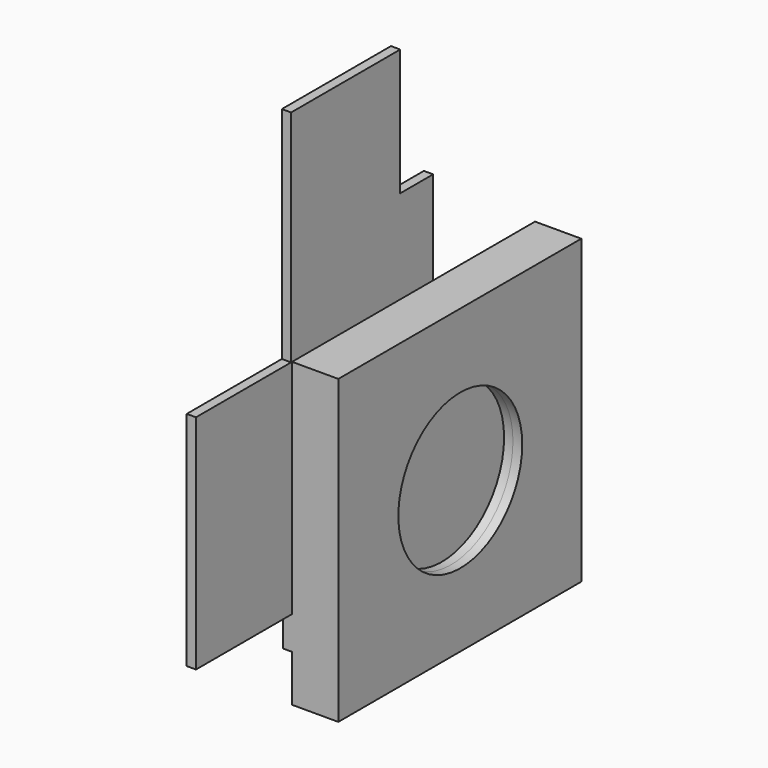
from build123d import *

# Parameters (mm, degrees)
F0_W      = 227.177798748
F0_H      = 67.4825310707
F0_W_2    = 7.6686143875
F0_W_3    = 40.7849550247
F0_H_2    = 19.1998630762
F1_DEPTH  = 25.4
F2_W      = 713.7889862061
F2_H      = 722.4479019642
F3_DEPTH  = 10751.3055801392
F5_W      = 833.6800336838
F5_H      = 828.9024829865
F6_DEPTH  = 25.4
F7_W      = 833.6800336838
F7_H      = 828.9024829865
F7_R      = 213.8106585198
F8_DEPTH  = 25.4
F9_W      = 805.6761920452
F9_H      = 828.9024829865
F9_R      = 212.5191058953
F9_W_2    = 28.0038416386
F10_DEPTH = 25.4
F11_W     = 833.6800336838
F11_H     = 828.9024829865
F11_R     = 151.5456161356
F12_DEPTH = 25.4
F13_W     = 680.4287135601
F13_H     = 667.77536273
F13_R     = 210.9258695705
F14_DEPTH = 25.4
F15_W     = 153.2513201237
F15_H     = 667.77536273
F16_DEPTH = 25.4
F17_W     = 371.1061030626
F17_H     = 256.3967704773
F17_W_2   = 32.0261418819
F17_H_2   = 25.0417590141
F17_W_3   = 119.3500384688
F17_H_3   = 111.177533865
F18_DEPTH = 25.4


with BuildPart() as f1:
    # F0 (on Right) → F1 (new body)
    with BuildSketch(Plane.YZ):
        Polygon((-598.1872081757, 183.7075799704), (-598.1872081757, 196.1238980293), (-605.8558225632, 196.1238980293), (-605.8558225632, 145.6781327724), (-598.1872081757, 145.6781327724), align=None)
        Polygon((-605.8558225632, 196.1238980293), (-598.1872081757, 196.1238980293), (-598.1872081757, 401.8925428391), (-605.8558225632, 401.8925428391), (-605.8558225632, 215.3237611055), align=None)
        Polygon((-1197.3617076874, 196.1238980293), (-605.8558225632, 196.1238980293), (-605.8558225632, 215.3237611055), (-1548.1258630753, 215.3237611055), (-1548.1258630753, 196.1238980293), align=None)
        Polygon((698.481798172, 183.7075799704), (-598.1872081757, 183.7075799704), (-598.1872081757, 145.6781327724), (-598.1872081757, 78.1956017017), (-598.1872081757, 8.7382793427), (698.481798172, 8.7382793427), align=None)
        Polygon((-1197.3617076874, 145.6781327724), (-1197.3617076874, 196.1238980293), (-1548.1258630753, 196.1238980293), (-1548.1258630753, 78.1956017017), (-833.0336213112, 78.1956017017), (-833.0336213112, 145.6781327724), align=None)
        with Locations((-719.4447219372, 111.9368672371)):
            Rectangle(F0_W, F0_H)
        with Locations((-602.0215153694, 111.9368672371)):
            Rectangle(F0_W_2, F0_H)
        Polygon((-1548.1258630753, 215.3237611055), (-605.8558225632, 215.3237611055), (-605.8558225632, 401.8925428391), (-1588.9108181, 401.8925428391), (-1588.9108181, 215.3237611055), align=None)
        with Locations((-1568.5183405876, 205.7238295674)):
            Rectangle(F0_W_3, F0_H_2)
    extrude(amount=F1_DEPTH)

    # F2 (on face) → F3 (join)
    with BuildSketch(Plane(origin=(0, 0, 0), x_dir=(0, -1, 0), z_dir=(-1, 0, 0))):
        with Locations((448.7802386284, 201.1957615614)):
            Rectangle(F2_W, F2_H)
    extrude(amount=F3_DEPTH)


with BuildPart() as f6:
    # F5 (on Right) → F6 (new body)
    with BuildSketch(Plane.YZ):
        with Locations((-1.6488134861, 0.6756186485)):
            Rectangle(F5_W, F5_H)
    extrude(amount=F6_DEPTH)

    # F7 (on face) → F8 (join)
    with BuildSketch(Plane.YZ.offset(25.4)):
        with Locations((-1.6488134861, 0.6756186485)):
            Rectangle(F7_W, F7_H)
        Circle(F7_R, mode=Mode.SUBTRACT)
    extrude(amount=F8_DEPTH)

    # F9 (on face) → F10 (join)
    with BuildSketch(Plane.YZ.offset(50.8)):
        with Locations((-15.6507343054, 0.6756186485)):
            Rectangle(F9_W, F9_H)
        Circle(F9_R, mode=Mode.SUBTRACT)
        with Locations((401.1892825365, 0.6756186485)):
            Rectangle(F9_W_2, F9_H)
    extrude(amount=F10_DEPTH)

    # F11 (on face) → F12 (join)
    with BuildSketch(Plane(origin=(0, 0, 0), x_dir=(0, -1, 0), z_dir=(-1, 0, 0))):
        with Locations((1.6488134861, 0.6756186485)):
            Rectangle(F11_W, F11_H)
        Circle(F11_R, mode=Mode.SUBTRACT)
    extrude(amount=F12_DEPTH)

    # F13 (on face) → F14 (join)
    with BuildSketch(Plane(origin=(-25.4, 0, 0), x_dir=(0, -1, 0), z_dir=(-1, 0, 0))):
        with Locations((-74.9768465757, -79.8879414797)):
            Rectangle(F13_W, F13_H)
        Circle(F13_R, mode=Mode.SUBTRACT)
    extrude(amount=F14_DEPTH)

    # F15 (on face) → F16 (join)
    with BuildSketch(Plane(origin=(-25.4, 0, 0), x_dir=(0, -1, 0), z_dir=(-1, 0, 0))):
        Polygon((418.488830328, 415.1268601418), (-415.1912033558, 415.1268601418), (-415.1912033558, 253.9997398853), (265.2375102043, 253.9997398853), (418.488830328, 253.9997398853), align=None)
        with Locations((341.8631702662, -79.8879414797)):
            Rectangle(F15_W, F15_H)
    extrude(amount=F16_DEPTH)

    # F17 (on face) → F18 (join)
    with BuildSketch(Plane(origin=(-50.8, 0, 0), x_dir=(0, -1, 0), z_dir=(-1, 0, 0))):
        with Locations((232.9357787967, 543.3252453804)):
            Rectangle(F17_W, F17_H)
        Polygon((418.488830328, 415.1268601418), (47.3827272654, 415.1268601418), (47.3827272654, 671.523630619), (-65.5413940549, 671.523630619), (-65.5413940549, 168.3508753777), (-65.5413940549, 57.1733415127), (-65.5413940549, -285.7585549355), (418.488830328, -285.7585549355), (418.488830328, -220.9893465042), (418.488830328, -194.4699287415), (418.488830328, 0.6756186485), align=None)
        with Locations((16.013070941, -182.512909174)):
            Rectangle(F17_W_2, F17_H_2, mode=Mode.SUBTRACT)
        Polygon((418.488830328, 671.523630619), (418.488830328, 415.1268601418), (421.7643141747, 415.1268601418), (421.7643141747, 1019.0404653549), (47.3827272654, 1019.0404653549), (47.3827272654, 671.523630619), align=None)
        Polygon((421.7643141747, 415.1268601418), (418.488830328, 415.1268601418), (418.488830328, 0.6756186485), (418.488830328, -194.4699287415), (748.2059001923, -194.4699287415), (748.2059001923, 415.1268601418), align=None)
        with Locations((-125.2164132893, 112.7621084452)):
            Rectangle(F17_W_3, F17_H_3)
    extrude(amount=F18_DEPTH)


solid = f6.part
